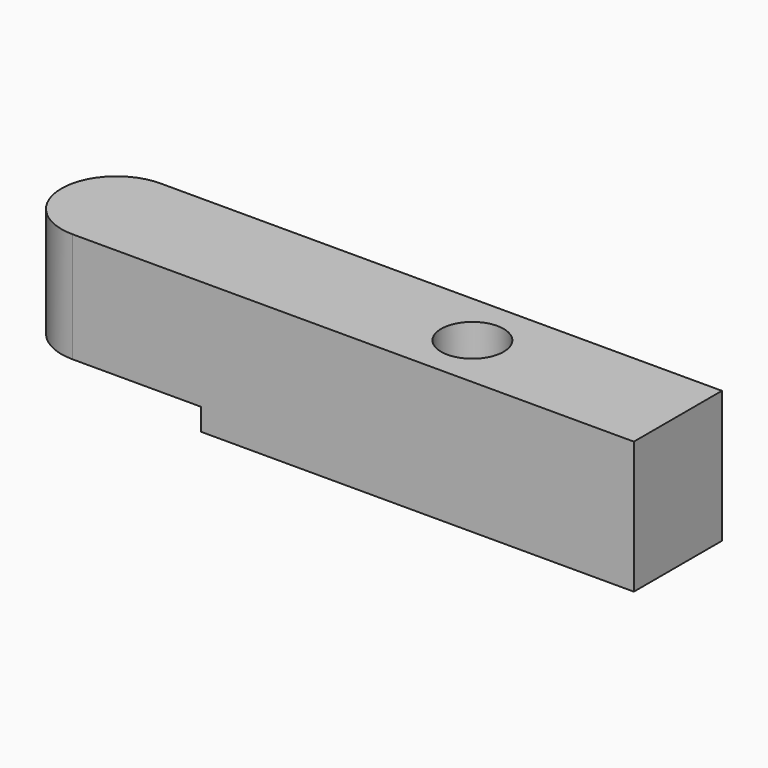
from build123d import *

# Parameters (mm, degrees)
F0_W     = 84
F0_H     = 15
F1_DEPTH = 15
F3_R     = 7.49999
F4_W     = 59
F4_H     = 15
F5_DEPTH = 3
F2_R     = 4.25
F6_DEPTH = 18.001


# Not quite as in the source:
# - a fillet or chamfer is up to 0.001 mm smaller than in the source, because OpenCascade refuses the exact size


with BuildPart() as f1:
    # F0 (on Front) → F1 (new body)
    with BuildSketch(Plane.XZ):
        Rectangle(F0_W, F0_H)
    extrude(amount=-F1_DEPTH)

    # F3 (radius 7.5 in the source; OpenCascade refuses exactly that, so slightly less here)
    f3_edges = [f1.edges().sort_by_distance(p)[0] for p in [
        (-42, 15, 0),
        (-42, 0, 0),
    ]]
    fillet(f3_edges, radius=F3_R)

    # F4 (on face) → F5 (join)
    with BuildSketch(Plane(origin=(0, 0, -7.5), x_dir=(1, 0, 0), z_dir=(0, 0, -1))):
        with Locations((12.5, -7.5)):
            Rectangle(F4_W, F4_H)
    extrude(amount=F5_DEPTH)

    # F2 (on face) → F6 (cut, through all)
    with BuildSketch(Plane.XY.offset(7.5)):
        with Locations((14, 7.5)):
            Circle(F2_R)
    extrude(amount=-F6_DEPTH, mode=Mode.SUBTRACT)


solid = f1.part
